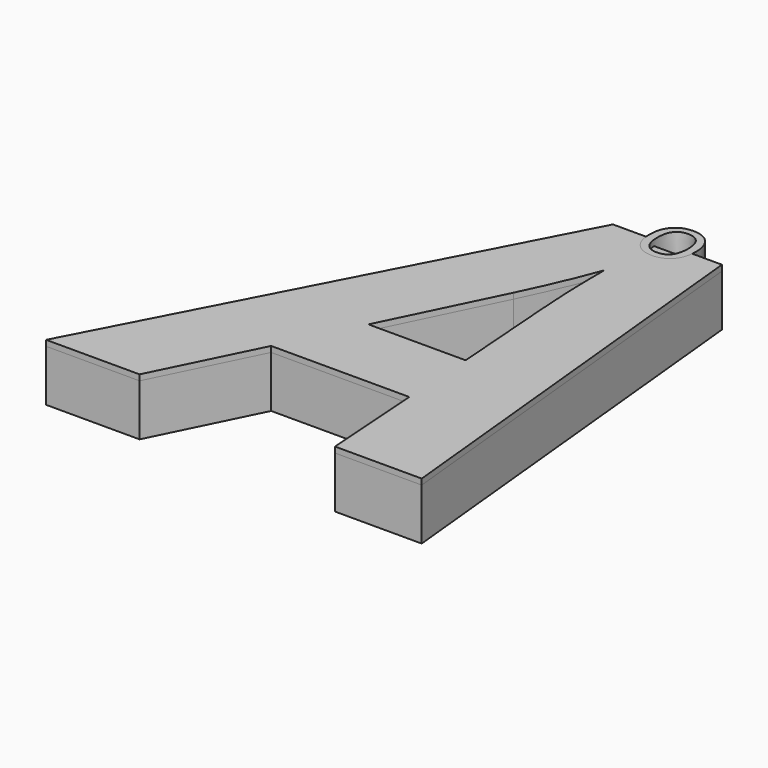
from build123d import *

# Parameters (mm, degrees)
F0_TEXT_SIZE = 66.3711999853
F1_DEPTH     = 5.715
F2_TEXT_SIZE = 10.5214373131
F3_DEPTH     = 6.35
F4_DEPTH     = 0.635


# Not quite as in the source:
# - Text() gives the source's letters only with a copy of the font that has no kerning and outlines rounded to 1/6400 em; it was checked with that copy


with BuildPart() as f1:
    # F0 (on Top) → F1 (new body)
    with BuildSketch(Plane.XY):
        with Locations((0, -47.7872639894)):
            Text('A', F0_TEXT_SIZE, font='Open Sans', font_style=FontStyle.BOLDITALIC, text_align=(TextAlign.LEFT, TextAlign.BOTTOM))
    extrude(amount=F1_DEPTH)

    # F2 (on Top) → F3 (join)
    with BuildSketch(Plane.XY):
        with Locations((23.8964129239, -2.5471986737)):
            Text('o', F2_TEXT_SIZE, font='Open Sans', text_align=(TextAlign.LEFT, TextAlign.BOTTOM))
    extrude(amount=F3_DEPTH)

    # F4 (add): a face of the model
    f4_faces = [f1.faces().sort_by_distance(p)[0] for p in [
        (8.9868022303, -24.2898228187, 5.715),
    ]]
    extrude(f4_faces, amount=F4_DEPTH)


solid = f1.part
